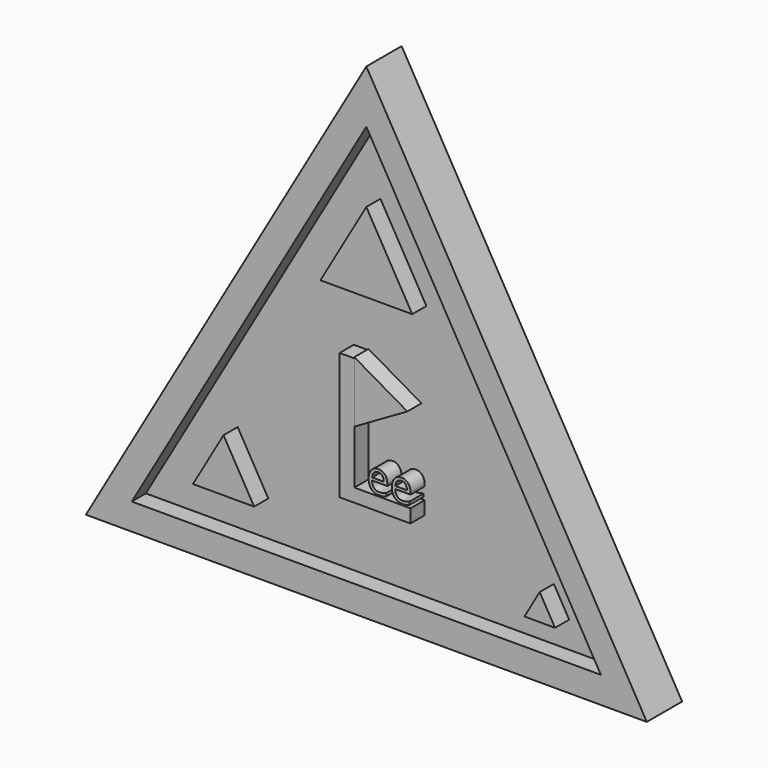
from build123d import *

# Parameters (mm, degrees)
F0_TEXT_SIZE = 4.6735796699
F1_DEPTH     = 5
F2_DEPTH     = 3


# Not quite as in the source:
# - Text() gives the source's letters only with a copy of the font that has no kerning and outlines rounded to 1/6400 em; it was checked with that copy


with BuildPart() as f1:
    # F0 (on Front) → F1 (new body)
    with BuildSketch(Plane.XZ):
        Polygon((31.7542648054, 0), (0, 55), (-31.7542648054, 0), align=None)
        Polygon((-26.5581123827, 3), (0, 49), (26.5581123827, 3), align=None, mode=Mode.SUBTRACT)
        Polygon((-5.1961524227, 32), (5.1961524227, 32), (0, 41), align=None)
        Polygon((-12.7017059222, 7), (-16.1658075373, 13), (-19.6299091524, 7), align=None)
        Polygon((17.8978583449, 6), (21.36195996, 6), (19.6299091524, 9), align=None)
        Polygon((-1.3496062992, 18.6667503362), (4.6418593326, 22.1259246316), (-1.3581406674, 25.5900262467), (-1.3581406674, 25.467191601), (-1.3496062992, 25.467191601), align=None)
        Polygon((-1.3496062992, 12.5916010499), (-1.3496062992, 18.6667503362), (-1.3581406674, 18.6618230164), (-1.3581406674, 25.467191601), (-3.0220472441, 25.467191601), (-3.0220472441, 11.0766404199), (5, 11.0766404199), (5, 12.5916010499), align=None)
        with Locations((0, 12.7685871024)):
            Text('ee', F0_TEXT_SIZE, font='Open Sans', text_align=(TextAlign.LEFT, TextAlign.BOTTOM))
    extrude(amount=F1_DEPTH)


with BuildPart() as f2:
    # F0 (on Front) → F2 (new body)
    with BuildSketch(Plane.XZ):
        Polygon((26.5581123827, 3), (0, 49), (-26.5581123827, 3), align=None)
        Polygon((-19.6299091524, 7), (-16.1658075373, 13), (-12.7017059222, 7), align=None, mode=Mode.SUBTRACT)
        Polygon((19.6299091524, 9), (21.36195996, 6), (17.8978583449, 6), align=None, mode=Mode.SUBTRACT)
        with BuildLine():
            add(Edge.make_bspline(
                [(1.8906090259, 12.7605543874), (1.7116985541, 12.7225815526), (1.4583029064, 12.7225815526)],
                knots=[0, 0, 0, 1, 1, 1], degree=2))
            add(Edge.make_bspline(
                [(1.4583029064, 12.7225815526), (0.9040455674, 12.7225815526), (0.5831020885, 13.0606858318)],
                knots=[0, 0, 0, 1, 1, 1], degree=2))
            add(Edge.make_bspline(
                [(0.5831020885, 13.0606858318), (0.2621586096, 13.398790111), (0.2621586096, 13.9983227531)],
                knots=[0, 0, 0, 1, 1, 1], degree=2))
            add(Edge.make_bspline(
                [(0.2621586096, 13.9983227531), (0.2621586096, 14.6036973697), (0.5600993136, 14.9596926961)],
                knots=[0, 0, 0, 1, 1, 1], degree=2))
            add(Edge.make_bspline(
                [(0.5600993136, 14.9596926961), (0.8580400175, 15.3156880225), (1.360449832, 15.3156880225)],
                knots=[0, 0, 0, 1, 1, 1], degree=2))
            add(Edge.make_bspline(
                [(1.360449832, 15.3156880225), (1.8299985395, 15.3156880225), (2.1038410983, 15.0064284928)],
                knots=[0, 0, 0, 1, 1, 1], degree=2))
            add(Edge.make_bspline(
                [(2.1038410983, 15.0064284928), (2.3776836571, 14.6971689631), (2.3776836571, 14.1903776676)],
                knots=[0, 0, 0, 1, 1, 1], degree=2))
            Line((2.3776836571, 14.1903776676), (2.3776836571, 13.9508567096))
            Line((2.3776836571, 13.9508567096), (0.6550314006, 13.9508567096))
            add(Edge.make_bspline(
                [(0.6550314006, 13.9508567096), (0.6667153498, 13.510517875), (0.8777566818, 13.2823157427)],
                knots=[0, 0, 0, 1, 1, 1], degree=2))
            add(Edge.make_bspline(
                [(0.8777566818, 13.2823157427), (1.0887980137, 13.0541136104), (1.472177596, 13.0541136104)],
                knots=[0, 0, 0, 1, 1, 1], degree=2))
            add(Edge.make_bspline(
                [(1.472177596, 13.0541136104), (1.8760040894, 13.0541136104), (2.270337374, 13.2228006266)],
                knots=[0, 0, 0, 1, 1, 1], degree=2))
            Line((2.270337374, 13.2228006266), (2.270337374, 12.8846963474))
            add(Edge.make_bspline(
                [(2.270337374, 12.8846963474), (2.0695194976, 12.7985272222), (1.8906090259, 12.7605543874)],
                knots=[0, 0, 0, 1, 1, 1], degree=2))
        make_face(mode=Mode.SUBTRACT)
        with BuildLine():
            add(Edge.make_bspline(
                [(4.5129253688, 12.7605543874), (4.334014897, 12.7225815526), (4.0806192493, 12.7225815526)],
                knots=[0, 0, 0, 1, 1, 1], degree=2))
            add(Edge.make_bspline(
                [(4.0806192493, 12.7225815526), (3.5263619103, 12.7225815526), (3.2054184314, 13.0606858318)],
                knots=[0, 0, 0, 1, 1, 1], degree=2))
            add(Edge.make_bspline(
                [(3.2054184314, 13.0606858318), (2.8844749525, 13.398790111), (2.8844749525, 13.9983227531)],
                knots=[0, 0, 0, 1, 1, 1], degree=2))
            add(Edge.make_bspline(
                [(2.8844749525, 13.9983227531), (2.8844749525, 14.6036973697), (3.1824156565, 14.9596926961)],
                knots=[0, 0, 0, 1, 1, 1], degree=2))
            add(Edge.make_bspline(
                [(3.1824156565, 14.9596926961), (3.4803563604, 15.3156880225), (3.982766175, 15.3156880225)],
                knots=[0, 0, 0, 1, 1, 1], degree=2))
            add(Edge.make_bspline(
                [(3.982766175, 15.3156880225), (4.4523148824, 15.3156880225), (4.7261574412, 15.0064284928)],
                knots=[0, 0, 0, 1, 1, 1], degree=2))
            add(Edge.make_bspline(
                [(4.7261574412, 15.0064284928), (5, 14.6971689631), (5, 14.1903776676)],
                knots=[0, 0, 0, 1, 1, 1], degree=2))
            Line((5, 14.1903776676), (5, 13.9508567096))
            Line((5, 13.9508567096), (3.2773477435, 13.9508567096))
            add(Edge.make_bspline(
                [(3.2773477435, 13.9508567096), (3.2890316927, 13.510517875), (3.5000730247, 13.2823157427)],
                knots=[0, 0, 0, 1, 1, 1], degree=2))
            add(Edge.make_bspline(
                [(3.5000730247, 13.2823157427), (3.7111143567, 13.0541136104), (4.094493939, 13.0541136104)],
                knots=[0, 0, 0, 1, 1, 1], degree=2))
            add(Edge.make_bspline(
                [(4.094493939, 13.0541136104), (4.4983204323, 13.0541136104), (4.892653717, 13.2228006266)],
                knots=[0, 0, 0, 1, 1, 1], degree=2))
            Line((4.892653717, 13.2228006266), (4.892653717, 12.8846963474))
            add(Edge.make_bspline(
                [(4.892653717, 12.8846963474), (4.6918358405, 12.7985272222), (4.5129253688, 12.7605543874)],
                knots=[0, 0, 0, 1, 1, 1], degree=2))
        make_face(mode=Mode.SUBTRACT)
        Polygon((-1.3581406674, 25.5900262467), (4.6418593326, 22.1259246316), (-1.3496062992, 18.6667503362), (-1.3496062992, 12.5916010499), (5, 12.5916010499), (5, 11.0766404199), (-3.0220472441, 11.0766404199), (-3.0220472441, 25.467191601), (-1.3581406674, 25.467191601), align=None, mode=Mode.SUBTRACT)
        Polygon((0, 41), (5.1961524227, 32), (-5.1961524227, 32), align=None, mode=Mode.SUBTRACT)
    extrude(amount=F2_DEPTH)


solid = Compound([f1.part, f2.part])
